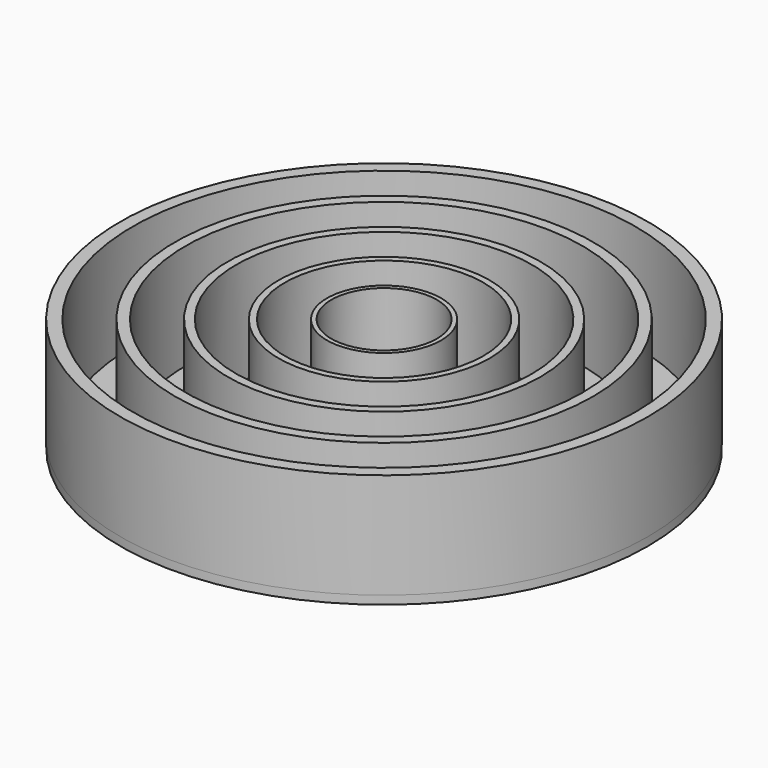
from build123d import *

# Parameters (mm, degrees)
F0_R         = 25
F1_DEPTH     = 0.8
F2_R         = 25.01
F2_R_2       = 23.81
F2_R_3       = 19.81
F2_R_4       = 18.81
F2_R_5       = 14.81
F2_R_6       = 14.01
F2_R_7       = 10.01
F2_R_8       = 9.41
F2_R_9       = 5.41
F2_R_10      = 5
F3_DEPTH     = 10
F4_TEXT_SIZE = 2.4623381953
F5_DEPTH     = 2


# Not quite as in the source:
# - Text() gives the source's letters only with a copy of the font that has no kerning and outlines rounded to 1/6400 em; it was checked with that copy


with BuildPart() as f1:
    # F0 (on Top) → F1 (new body)
    with BuildSketch(Plane.XY):
        Circle(F0_R)
    extrude(amount=F1_DEPTH)

    # F2 (on face) → F3 (join)
    with BuildSketch(Plane.XY.offset(0.8)):
        Circle(F2_R)
        Circle(F2_R_2, mode=Mode.SUBTRACT)
        Circle(F2_R_3)
        Circle(F2_R_4, mode=Mode.SUBTRACT)
        Circle(F2_R_5)
        Circle(F2_R_6, mode=Mode.SUBTRACT)
        Circle(F2_R_7)
        Circle(F2_R_8, mode=Mode.SUBTRACT)
        Circle(F2_R_9)
        Circle(F2_R_10, mode=Mode.SUBTRACT)
    extrude(amount=F3_DEPTH)

    # F4 (on Top) → F5 (join)
    with BuildSketch(Plane.XY):
        with Locations((1, -0.4143339531)):
            Text('0.4  0.6  0.8  1.0  1.2', F4_TEXT_SIZE, font='Open Sans', text_align=(TextAlign.LEFT, TextAlign.BOTTOM))
    extrude(amount=F5_DEPTH)


solid = f1.part
